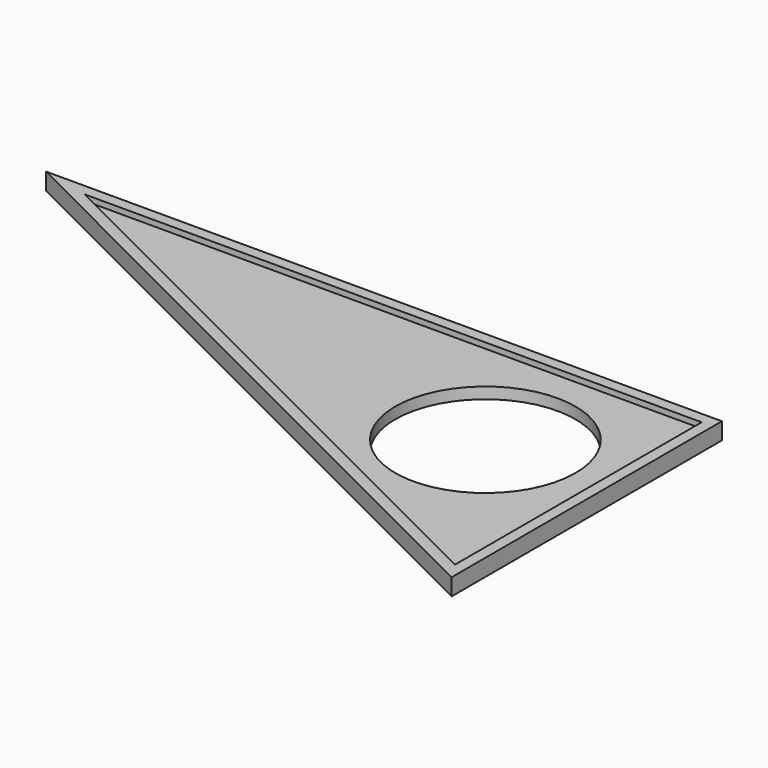
from build123d import *

# Parameters (mm, degrees)
F1_DEPTH = 3
F2_T     = -2
F4_DEPTH = 2.001


# Not quite as in the source:
# - ends of sketch curves that miss each other by under 0.0002 mm in the source are joined


with BuildPart() as f1:
    # F0 (on Top) → F1 (new body)
    with BuildSketch(Plane.XY):
        Polygon((0, -60), (0, 0), (-120, 0), align=None)
    extrude(amount=F1_DEPTH)

    # F2
    f2_openings = [f1.faces().sort_by_distance(p)[0] for p in [
        (-40, -20, 3),
    ]]
    offset(amount=F2_T, openings=f2_openings)

    # F3 (on face) → F4 (cut, through all)
    with BuildSketch(Plane.XY.offset(2)):
        with BuildLine():
            ThreePointArc((-12.0208152802, -12.0208152802), (-38.1165962993, -29.457458697), (-7.3345237792, -23.3345237792))
            ThreePointArc((-7.3345237792, -23.3345237792), (-8.552451259, -17.2115888613), (-12.0208152802, -12.0208152802))
        make_face()
    extrude(amount=-F4_DEPTH, mode=Mode.SUBTRACT)


solid = f1.part
